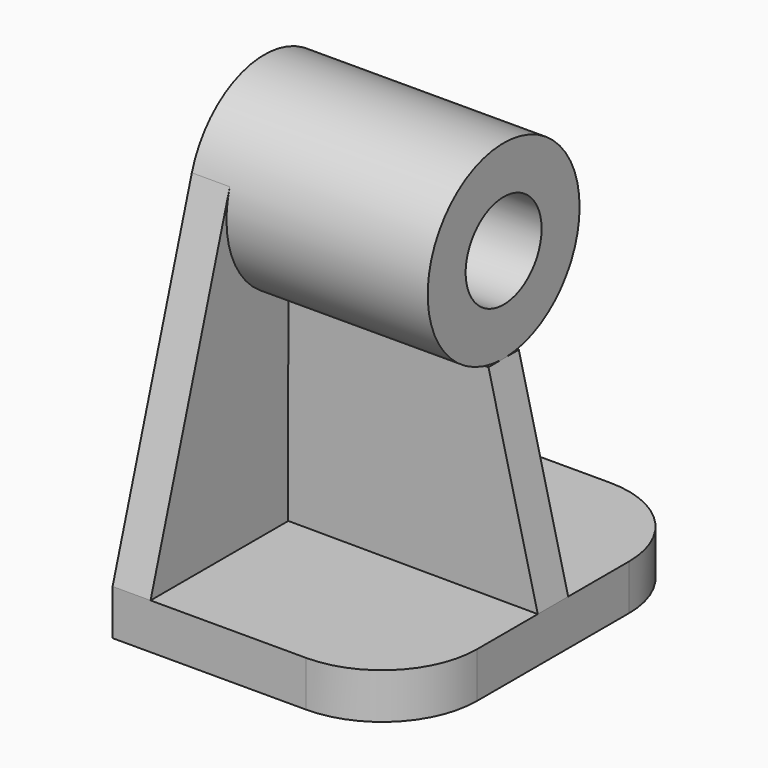
from build123d import *

# Parameters (mm, degrees)
F0_W      = 76
F0_H      = 100
F1_DEPTH  = 12
F2_R      = 25
F3_R      = 25
F4_DEPTH  = 25
F5_R      = 12.5
F6_DEPTH  = 63
F7_DEPTH  = 63
F8_R      = 12.5
F9_DEPTH  = 63.001
F11_DEPTH = 10
F13_DEPTH = 5


with BuildPart() as f1:
    # F0 (on Top) → F1 (new body)
    with BuildSketch(Plane.XY):
        Rectangle(F0_W, F0_H)
    extrude(amount=F1_DEPTH)

    # F2
    f2_edges = [f1.edges().sort_by_distance(p)[0] for p in [
        (38, -50, 6),
        (38, 50, 6),
    ]]
    fillet(f2_edges, radius=F2_R)

    # F5 (on face) → F6 (cut)
    with BuildSketch(Plane.YZ.offset(25)):
        with Locations((0, 90)):
            Circle(F5_R)
    extrude(amount=F6_DEPTH, mode=Mode.SUBTRACT)


with BuildPart() as f4:
    # F3 (on Right) → F4 (new body)
    with BuildSketch(Plane.YZ):
        with Locations((0, 90)):
            Circle(F3_R)
    extrude(amount=F4_DEPTH)

    # F7 (add): a face of the model
    f7_faces = [f4.faces().sort_by_distance(p)[0] for p in [
        (25, 0, 90),
    ]]
    extrude(f7_faces, amount=-F7_DEPTH)

    # F8 (on face) → F9 (cut, through all)
    with BuildSketch(Plane.YZ.offset(25)):
        with Locations((0, 90)):
            Circle(F8_R)
    extrude(amount=-F9_DEPTH, mode=Mode.SUBTRACT)

    # F10 (on face) → F11 (join)
    with BuildSketch(Plane(origin=(-38, 0, 0), x_dir=(0, -1, 0), z_dir=(-1, 0, 0))):
        with BuildLine():
            ThreePointArc((25, 90), (-3.6966549694, 65.2748156319), (-23.906779363, 97.3120380532))
            Line((-23.906779363, 97.3120380532), (-50, 12))
            Line((-50, 12), (50, 12))
            Line((50, 12), (23.906779363, 97.3120380532))
            ThreePointArc((23.906779363, 97.3120380532), (24.7251843681, 93.6966549694), (25, 90))
        make_face()
    extrude(amount=-F11_DEPTH)

    # F12 (on Front) → F13 (join, symmetric)
    with BuildSketch(Plane.XZ):
        Polygon((38, 12), (25, 65.0144964457), (-27.6728401392, 64.9104069279), (-27.8638396412, 12.2388377786), align=None)
    extrude(amount=F13_DEPTH, both=True)


solid = Compound([f1.part, f4.part])
